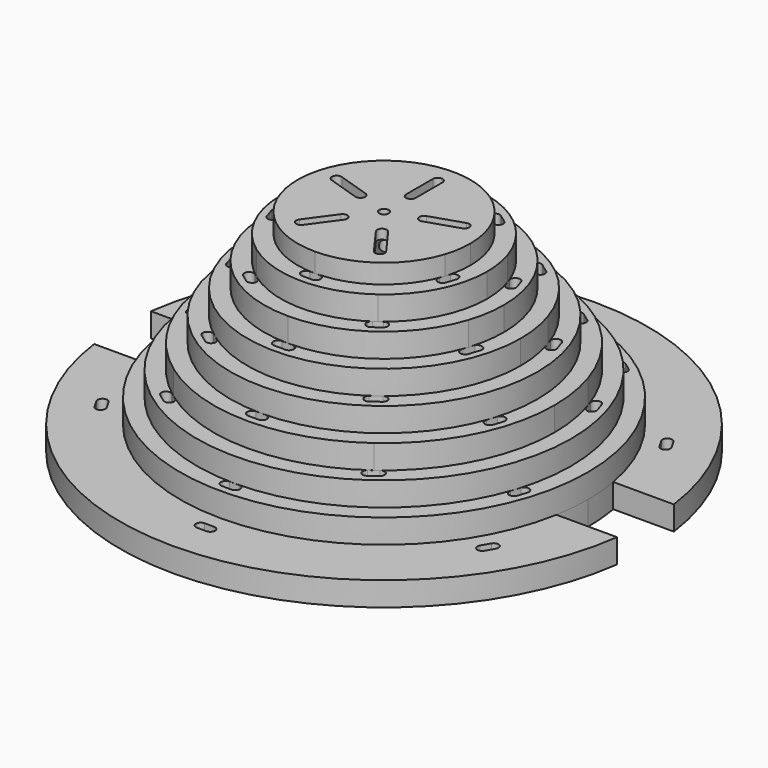
from build123d import *

# Parameters (mm, degrees)
F0_R      = 55
F1_DEPTH  = 5
F2_R      = 42.5
F3_DEPTH  = 5
F5_DEPTH  = 10.001
F7_DEPTH  = 5.001
F8_R      = 39
F9_DEPTH  = 5
F11_DEPTH = 15.001
F13_DEPTH = 5
F15_DEPTH = 20.001
F16_R     = 32
F17_DEPTH = 5
F19_DEPTH = 5
F21_DEPTH = 30.001
F22_DEPTH = 20.001
F24_DEPTH = 5
F26_DEPTH = 35.001
F28_DEPTH = 5
F30_DEPTH = 40.001
F32_DEPTH = 4
F33_R     = 1
F34_DEPTH = 44.001
F41_DEPTH = 5.0010001


with BuildPart() as f1:
    # F0 (on Top) → F1 (new body)
    with BuildSketch(Plane.XY):
        Circle(F0_R)
    extrude(amount=F1_DEPTH)

    # F2 (on face) → F3 (join)
    with BuildSketch(Plane.XY.offset(5)):
        Circle(F2_R)
    extrude(amount=F3_DEPTH)

    # F4 (on face) → F5 (cut, through all)
    with BuildSketch(Plane.XY.offset(10)):
        with BuildLine():
            Line((1, -39), (-1, -39))
            ThreePointArc((-1, -39), (-2, -40), (-1, -41))
            Line((-1, -41), (1, -41))
            ThreePointArc((1, -41), (2, -40), (1, -39))
        make_face()
        with BuildLine():
            Line((37.4002211299, -11.1006062643), (36.7821871411, -13.0027192969))
            ThreePointArc((36.7821871411, -13.0027192969), (37.4242266631, -14.2627928076), (38.6843001737, -13.6207532857))
            Line((38.6843001737, -13.6207532857), (39.3023341625, -11.7186402531))
            ThreePointArc((39.3023341625, -11.7186402531), (38.6602946406, -10.4585667424), (37.4002211299, -11.1006062643))
        make_face()
        with BuildLine():
            Line((22.114607845, 32.1394480329), (23.7326418338, 30.9638775283))
            ThreePointArc((23.7326418338, 30.9638775283), (25.1294440804, 31.1851092704), (24.9082123384, 32.5819115171))
            Line((24.9082123384, 32.5819115171), (23.2901783496, 33.7574820217))
            ThreePointArc((23.2901783496, 33.7574820217), (21.8933761029, 33.5362502796), (22.114607845, 32.1394480329))
        make_face()
        with BuildLine():
            Line((-23.7326418338, 30.9638775283), (-22.114607845, 32.1394480329))
            ThreePointArc((-22.114607845, 32.1394480329), (-21.8933761029, 33.5362502796), (-23.2901783496, 33.7574820217))
            Line((-23.2901783496, 33.7574820217), (-24.9082123384, 32.5819115171))
            ThreePointArc((-24.9082123384, 32.5819115171), (-25.1294440804, 31.1851092704), (-23.7326418338, 30.9638775283))
        make_face()
        with BuildLine():
            Line((-36.7821871411, -13.0027192969), (-37.4002211299, -11.1006062643))
            ThreePointArc((-37.4002211299, -11.1006062643), (-38.6602946406, -10.4585667424), (-39.3023341625, -11.7186402531))
            Line((-39.3023341625, -11.7186402531), (-38.6843001737, -13.6207532857))
            ThreePointArc((-38.6843001737, -13.6207532857), (-37.4242266631, -14.2627928076), (-36.7821871411, -13.0027192969))
        make_face()
    extrude(amount=-F5_DEPTH, mode=Mode.SUBTRACT)

    # F6 (on face) → F7 (cut, through all)
    with BuildSketch(Plane.XY.offset(5)):
        with BuildLine():
            ThreePointArc((-1, 47.5), (-2, 46.5), (-1, 45.5))
            Line((-1, 45.5), (1, 45.5))
            ThreePointArc((1, 45.5), (2, 46.5), (1, 47.5))
            Line((1, 47.5), (-1, 47.5))
        make_face()
        with BuildLine():
            Line((-40.6362066798, 24.6160254038), (-41.6362066798, 22.8839745962))
            ThreePointArc((-41.6362066798, 22.8839745962), (-41.270181276, 21.5179491924), (-39.9041558722, 21.8839745962))
            Line((-39.9041558722, 21.8839745962), (-38.9041558722, 23.6160254038))
            ThreePointArc((-38.9041558722, 23.6160254038), (-39.270181276, 24.9820508076), (-40.6362066798, 24.6160254038))
        make_face()
        with BuildLine():
            Line((-41.6362066798, -22.8839745962), (-40.6362066798, -24.6160254038))
            ThreePointArc((-40.6362066798, -24.6160254038), (-39.270181276, -24.9820508076), (-38.9041558722, -23.6160254038))
            Line((-38.9041558722, -23.6160254038), (-39.9041558722, -21.8839745962))
            ThreePointArc((-39.9041558722, -21.8839745962), (-41.270181276, -21.5179491924), (-41.6362066798, -22.8839745962))
        make_face()
        with BuildLine():
            Line((-1, -47.5), (1, -47.5))
            ThreePointArc((1, -47.5), (2, -46.5), (1, -45.5))
            Line((1, -45.5), (-1, -45.5))
            ThreePointArc((-1, -45.5), (-2, -46.5), (-1, -47.5))
        make_face()
        with BuildLine():
            Line((40.6362066798, -24.6160254038), (41.6362066798, -22.8839745962))
            ThreePointArc((41.6362066798, -22.8839745962), (41.270181276, -21.5179491924), (39.9041558722, -21.8839745962))
            Line((39.9041558722, -21.8839745962), (38.9041558722, -23.6160254038))
            ThreePointArc((38.9041558722, -23.6160254038), (39.270181276, -24.9820508076), (40.6362066798, -24.6160254038))
        make_face()
        with BuildLine():
            Line((41.6362066798, 22.8839745962), (40.6362066798, 24.6160254038))
            ThreePointArc((40.6362066798, 24.6160254038), (39.270181276, 24.9820508076), (38.9041558722, 23.6160254038))
            Line((38.9041558722, 23.6160254038), (39.9041558722, 21.8839745962))
            ThreePointArc((39.9041558722, 21.8839745962), (41.270181276, 21.5179491924), (41.6362066798, 22.8839745962))
        make_face()
    extrude(amount=-F7_DEPTH, mode=Mode.SUBTRACT)

    # F8 (on face) → F9 (join)
    with BuildSketch(Plane.XY.offset(10)):
        Circle(F8_R)
    extrude(amount=F9_DEPTH)

    # F10 (on face) → F11 (cut, through all)
    with BuildSketch(Plane.XY.offset(15)):
        with BuildLine():
            ThreePointArc((1, 35.5), (2, 36.5), (1, 37.5))
            Line((1, 37.5), (-1, 37.5))
            ThreePointArc((-1, 37.5), (-2, 36.5), (-1, 35.5))
            Line((-1, 35.5), (1, 35.5))
        make_face()
        with BuildLine():
            ThreePointArc((-33.4534893341, 11.9211598166), (-34.095528856, 13.1812333273), (-35.3556023667, 12.5391938054))
            Line((-35.3556023667, 12.5391938054), (-35.9736363554, 10.6370807728))
            ThreePointArc((-35.9736363554, 10.6370807728), (-35.3315968335, 9.3770072621), (-34.0715233229, 10.019046784))
            Line((-34.0715233229, 10.019046784), (-33.4534893341, 11.9211598166))
        make_face()
        with BuildLine():
            ThreePointArc((-21.6753934508, -28.132318048), (-23.0721956974, -28.3535497901), (-22.8509639553, -29.7503520368))
            Line((-22.8509639553, -29.7503520368), (-21.2329299666, -30.9259225414))
            ThreePointArc((-21.2329299666, -30.9259225414), (-19.8361277199, -30.7046907993), (-20.057359462, -29.3078885526))
            Line((-20.057359462, -29.3078885526), (-21.6753934508, -28.132318048))
        make_face()
        with BuildLine():
            ThreePointArc((20.057359462, -29.3078885526), (19.8361277199, -30.7046907993), (21.2329299666, -30.9259225414))
            Line((21.2329299666, -30.9259225414), (22.8509639553, -29.7503520368))
            ThreePointArc((22.8509639553, -29.7503520368), (23.0721956974, -28.3535497901), (21.6753934508, -28.132318048))
            Line((21.6753934508, -28.132318048), (20.057359462, -29.3078885526))
        make_face()
        with BuildLine():
            ThreePointArc((34.0715233229, 10.019046784), (35.3315968335, 9.3770072621), (35.9736363554, 10.6370807728))
            Line((35.9736363554, 10.6370807728), (35.3556023667, 12.5391938054))
            ThreePointArc((35.3556023667, 12.5391938054), (34.095528856, 13.1812333273), (33.4534893341, 11.9211598166))
            Line((33.4534893341, 11.9211598166), (34.0715233229, 10.019046784))
        make_face()
    extrude(amount=-F11_DEPTH, mode=Mode.SUBTRACT)

    # F12 (on face) → F13 (join)
    with BuildSketch(Plane.XY.offset(15)):
        with BuildLine():
            ThreePointArc((20.8663763999, -28.7201033414), (31.6307315928, -16.1166627719), (35.5, 0))
            ThreePointArc((35.5, 0), (35.0629360728, 5.5534236244), (33.7625062562, 10.9701035227))
            ThreePointArc((33.7625062562, 10.9701035227), (20.8663763618, 28.720103369), (0, 35.5))
            ThreePointArc((0, 35.5), (-20.8663763618, 28.720103369), (-33.7625062562, 10.9701035227))
            ThreePointArc((-33.7625062562, 10.9701035227), (-33.7625063538, -10.9701032224), (-20.8663763999, -28.7201033414))
            ThreePointArc((-20.8663763999, -28.7201033414), (0, -35.5), (20.8663763999, -28.7201033414))
        make_face()
    extrude(amount=F13_DEPTH)

    # F14 (on face) → F15 (cut, through all)
    with BuildSketch(Plane.XY.offset(20)):
        with BuildLine():
            ThreePointArc((0.9018983435, -34), (2, -33.0981016565), (1.0981016565, -32))
            Line((1.0981016565, -32), (-1.0981016565, -32))
            ThreePointArc((-1.0981016565, -32), (-2.0981016565, -33), (-1.0981016565, -34))
            Line((-1.0981016565, -34), (0.9018983435, -34))
        make_face()
        with BuildLine():
            ThreePointArc((32.6146234694, -9.6488215121), (32.0961992461, -8.3257628608), (30.7731405948, -8.8441870841))
            Line((30.7731405948, -8.8441870841), (30.094476448, -10.9329005559))
            ThreePointArc((30.094476448, -10.9329005559), (30.73651597, -12.1929740666), (31.9965894806, -11.5509345447))
            Line((31.9965894806, -11.5509345447), (32.6146234694, -9.6488215121))
        make_face()
        with BuildLine():
            ThreePointArc((19.2550474908, 28.0367003541), (17.8365420438, 27.9524972262), (17.9207451717, 26.5339917792))
            Line((17.9207451717, 26.5339917792), (19.697510975, 25.2430958608))
            ThreePointArc((19.697510975, 25.2430958608), (21.0943132217, 25.4643276029), (20.8730814796, 26.8611298496))
            Line((20.8730814796, 26.8611298496), (19.2550474908, 28.0367003541))
        make_face()
        with BuildLine():
            ThreePointArc((-20.7143496651, 26.9764552634), (-21.0726100213, 25.6013562171), (-19.697510975, 25.2430958608))
            Line((-19.697510975, 25.2430958608), (-17.9207451717, 26.5339917792))
            ThreePointArc((-17.9207451717, 26.5339917792), (-17.6995134296, 27.9307940259), (-19.0963156763, 28.1520257679))
            Line((-19.0963156763, 28.1520257679), (-20.7143496651, 26.9764552634))
        make_face()
        with BuildLine():
            ThreePointArc((-32.0572196387, -11.3643341054), (-30.8601312686, -12.129988926), (-30.094476448, -10.9329005559))
            Line((-30.094476448, -10.9329005559), (-30.7731405948, -8.8441870841))
            ThreePointArc((-30.7731405948, -8.8441870841), (-32.0332141055, -8.2021475621), (-32.6752536274, -9.4622210728))
            Line((-32.6752536274, -9.4622210728), (-32.0572196387, -11.3643341054))
        make_face()
    extrude(amount=-F15_DEPTH, mode=Mode.SUBTRACT)

    # F16 (on face) → F17 (join)
    with BuildSketch(Plane.XY.offset(20)):
        Circle(F16_R)
        with BuildLine():
            ThreePointArc((-15.8373506425, -23.721428586), (-15.6161189004, -25.1182308327), (-17.0129211471, -25.3394625748))
            Line((-17.0129211471, -25.3394625748), (-18.6309551359, -24.1638920702))
            ThreePointArc((-18.6309551359, -24.1638920702), (-19.0343579254, -22.7959428829), (-17.6664087381, -22.3925400934))
            Line((-17.6664087381, -22.3925400934), (-15.8373506425, -23.721428586))
        make_face(mode=Mode.SUBTRACT)
        with BuildLine():
            ThreePointArc((17.6664087381, -22.3925400934), (19.0632109848, -22.6137718354), (18.8419792427, -24.0105740821))
            Line((18.8419792427, -24.0105740821), (17.223945254, -25.1861445867))
            ThreePointArc((17.223945254, -25.1861445867), (15.7982899479, -25.1470838921), (15.8373506425, -23.721428586))
            Line((15.8373506425, -23.721428586), (17.6664087381, -22.3925400934))
        make_face(mode=Mode.SUBTRACT)
        with BuildLine():
            ThreePointArc((-27.454429727, 7.7318909655), (-28.7145032376, 7.0898514436), (-29.3565427596, 8.3499249542))
            Line((-29.3565427596, 8.3499249542), (-28.7385087708, 10.2520379868))
            ThreePointArc((-28.7385087708, 10.2520379868), (-27.5621700999, 11.0584163848), (-26.7557917018, 9.8820777139))
            Line((-26.7557917018, 9.8820777139), (-27.454429727, 7.7318909655))
        make_face(mode=Mode.SUBTRACT)
        with BuildLine():
            Line((-1.1304200705, 30.5), (0.8695799295, 30.5))
            ThreePointArc((0.8695799295, 30.5), (2, 29.6304200705), (1.1304200705, 28.5))
            Line((1.1304200705, 28.5), (-1.1304200705, 28.5))
            ThreePointArc((-1.1304200705, 28.5), (-2.1304200705, 29.5), (-1.1304200705, 30.5))
        make_face(mode=Mode.SUBTRACT)
        with BuildLine():
            ThreePointArc((26.7557917018, 9.8820777139), (27.3978312238, 11.1421512245), (28.6579047344, 10.5001117026))
            Line((28.6579047344, 10.5001117026), (29.2759387232, 8.59799867))
            ThreePointArc((29.2759387232, 8.59799867), (28.7982380774, 7.2541903197), (27.454429727, 7.7318909655))
            Line((27.454429727, 7.7318909655), (26.7557917018, 9.8820777139))
        make_face(mode=Mode.SUBTRACT)
    extrude(amount=F17_DEPTH)

    # F18 (on face) → F19 (join)
    with BuildSketch(Plane.XY.offset(25)):
        with BuildLine():
            ThreePointArc((16.751879483, -23.0569844903), (25.3936858812, -12.9387293567), (28.5, 0))
            ThreePointArc((28.5, 0), (28.1491177387, 4.458382053), (27.1051108399, 8.8069839534))
            ThreePointArc((27.1051108399, 8.8069839534), (16.7518798547, 23.0569842203), (0, 28.5))
            ThreePointArc((0, 28.5), (-16.7518798298, 23.0569842384), (-27.1051108209, 8.8069840118))
            ThreePointArc((-27.1051108209, 8.8069840118), (-27.1051106855, -8.8069844287), (-16.7518798178, -23.0569842471))
            ThreePointArc((-16.7518798178, -23.0569842471), (-2.069e-07, -28.5), (16.751879483, -23.0569844903))
        make_face()
    extrude(amount=F19_DEPTH)

    # F20 (on face) → F21 (cut, through all)
    with BuildSketch(Plane.XY.offset(30)):
        with BuildLine():
            ThreePointArc((0.7057068686, -27), (2, -26.2942931314), (1.2942931314, -25))
            Line((1.2942931314, -25), (-1.2942931314, -25))
            ThreePointArc((-1.2942931314, -25), (-2.2942931314, -26), (-1.2942931314, -27))
            Line((-1.2942931314, -27), (0.7057068686, -27))
        make_face()
        with BuildLine():
            Line((24.1763714807, -6.4944789427), (23.3764543341, -8.956370776))
            ThreePointArc((23.3764543341, -8.956370776), (24.018493856, -10.2164442867), (25.2785673666, -9.5744047648))
            Line((25.2785673666, -9.5744047648), (25.8966013554, -7.6722917322))
            ThreePointArc((25.8966013554, -7.6722917322), (25.6253928128, -6.2232704001), (24.1763714807, -6.4944789427))
        make_face()
        with BuildLine():
            Line((13.6475261683, 20.9861912742), (15.7417364464, 19.4646584446))
            ThreePointArc((15.7417364464, 19.4646584446), (17.138538693, 19.6858901866), (16.9173069509, 21.0826924333))
            Line((16.9173069509, 21.0826924333), (15.2992729622, 22.2582629379))
            ThreePointArc((15.2992729622, 22.2582629379), (13.8373637334, 22.448100503), (13.6475261683, 20.9861912742))
        make_face()
        with BuildLine():
            Line((-15.7417364464, 19.4646584446), (-13.6475261683, 20.9861912742))
            ThreePointArc((-13.6475261683, 20.9861912742), (-13.4262944262, 22.3829935208), (-14.8230966729, 22.6042252629))
            Line((-14.8230966729, 22.6042252629), (-16.4411306616, 21.4286547583))
            ThreePointArc((-16.4411306616, 21.4286547583), (-17.0734317109, 20.0969594938), (-15.7417364464, 19.4646584446))
        make_face()
        with BuildLine():
            Line((-23.3764543341, -8.956370776), (-24.1763714807, -6.4944789427))
            ThreePointArc((-24.1763714807, -6.4944789427), (-25.4364449914, -5.8524394208), (-26.0784845133, -7.1125129315))
            Line((-26.0784845133, -7.1125129315), (-25.4604505245, -9.0146259641))
            ThreePointArc((-25.4604505245, -9.0146259641), (-24.3893248353, -10.0274964653), (-23.3764543341, -8.956370776))
        make_face()
    extrude(amount=-F21_DEPTH, mode=Mode.SUBTRACT)

    # F22 (cut, through all): faces of the model
    f22_faces = [f1.faces().sort_by_distance(p)[0] for p in [
        (17.3875864045, -23.8314304164, 20),
        (28.0380968803, 9.1722603537, 20),
        (-0.0590895526, 29.5001990686, 20),
        (-28.0746162322, 9.0598653456, 20),
        (-17.2919775, -23.9008943515, 20),
    ]]
    extrude(f22_faces, amount=-F22_DEPTH, mode=Mode.SUBTRACT)

    # F23 (on face) → F24 (join)
    with BuildSketch(Plane.XY.offset(30)):
        with BuildLine():
            ThreePointArc((23.7764129613, -7.7254246936), (24.6922085285, -3.9108615399), (25, 0))
            ThreePointArc((25, 0), (22.2751630699, 11.3497625618), (14.6946311833, 20.2254249495))
            ThreePointArc((14.6946311833, 20.2254249495), (-7.01e-08, 25), (-14.6946312967, 20.2254248671))
            ThreePointArc((-14.6946312967, 20.2254248671), (-23.7764128803, 7.7254249427), (-23.7764129574, -7.7254247053))
            ThreePointArc((-23.7764129574, -7.7254247053), (-14.6946313729, -20.2254248118), (0, -25))
            ThreePointArc((0, -25), (14.6946313778, -20.2254248081), (23.7764129613, -7.7254246936))
        make_face()
    extrude(amount=F24_DEPTH)

    # F25 (on face) → F26 (cut, through all)
    with BuildSketch(Plane.XY.offset(35)):
        with BuildLine():
            ThreePointArc((0.8893935699, 21.5), (2, 22.3893935699), (1.1106064301, 23.5))
            Line((1.1106064301, 23.5), (-0.8893935699, 23.5))
            ThreePointArc((-0.8893935699, 23.5), (-1.8893935699, 22.5), (-0.8893935699, 21.5))
            Line((-0.8893935699, 21.5), (0.8893935699, 21.5))
        make_face()
        with BuildLine():
            Line((-22.006631872, 8.3181488502), (-22.6246658607, 6.4160358176))
            ThreePointArc((-22.6246658607, 6.4160358176), (-21.9826263388, 5.1559623069), (-20.7225528281, 5.7980018289))
            Line((-20.7225528281, 5.7980018289), (-20.1728773726, 7.4897289293))
            ThreePointArc((-20.1728773726, 7.4897289293), (-20.6755446618, 8.8208161394), (-22.006631872, 8.3181488502))
        make_face()
        with BuildLine():
            Line((-14.7114529049, -18.3591012871), (-13.0934189161, -19.5346717917))
            ThreePointArc((-13.0934189161, -19.5346717917), (-11.6966166695, -19.3134400496), (-11.9178484115, -17.9166378029))
            Line((-11.9178484115, -17.9166378029), (-13.356917437, -16.8710929552))
            ThreePointArc((-13.356917437, -16.8710929552), (-14.7781893369, -16.9378293872), (-14.7114529049, -18.3591012871))
        make_face()
        with BuildLine():
            Line((12.9144539529, -19.6646974485), (14.5324879416, -18.4891269439))
            ThreePointArc((14.5324879416, -18.4891269439), (14.7537196837, -17.0923246973), (13.356917437, -16.8710929552))
            Line((13.356917437, -16.8710929552), (11.9178484115, -17.9166378029))
            ThreePointArc((11.9178484115, -17.9166378029), (11.5421213594, -19.2889703964), (12.9144539529, -19.6646974485))
        make_face()
        with BuildLine():
            Line((22.6930243939, 6.2056498854), (22.0749904051, 8.107762918))
            ThreePointArc((22.0749904051, 8.107762918), (20.8149168945, 8.7498024399), (20.1728773726, 7.4897289293))
            Line((20.1728773726, 7.4897289293), (20.7225528281, 5.7980018289))
            ThreePointArc((20.7225528281, 5.7980018289), (21.9116126393, 5.0165900743), (22.6930243939, 6.2056498854))
        make_face()
    extrude(amount=-F26_DEPTH, mode=Mode.SUBTRACT)

    # F27 (on face) → F28 (join)
    with BuildSketch(Plane.XY.offset(35)):
        with BuildLine():
            ThreePointArc((12.6373831456, -17.3938652183), (19.1566403321, -9.7607956226), (21.5, 0))
            ThreePointArc((21.5, 0), (21.2352993391, 3.3633408951), (20.447715165, 6.6438651802))
            ThreePointArc((20.447715165, 6.6438651802), (12.6373830089, 17.3938653176), (0, 21.5))
            ThreePointArc((0, 21.5), (-12.637382926, 17.3938653778), (-20.4477151017, 6.643865375))
            ThreePointArc((-20.4477151017, 6.643865375), (-20.447715142, -6.643865251), (-12.6373831456, -17.3938652183))
            ThreePointArc((-12.6373831456, -17.3938652183), (0, -21.5), (12.6373831456, -17.3938652183))
        make_face()
    extrude(amount=F28_DEPTH)

    # F29 (on face) → F30 (cut, through all)
    with BuildSketch(Plane.XY.offset(40)):
        with BuildLine():
            ThreePointArc((-1, 47.5), (-2, 46.5), (-1, 45.5))
            Line((-1, 45.5), (1, 45.5))
            ThreePointArc((1, 45.5), (2, 46.5), (1, 47.5))
            Line((1, 47.5), (-1, 47.5))
        make_face()
        with BuildLine():
            ThreePointArc((-1.069542788, -18), (-2.069542788, -19), (-1.069542788, -20))
            Line((-1.069542788, -20), (0.930457212, -20))
            ThreePointArc((0.930457212, -20), (2, -19.069542788), (1.069542788, -18))
            Line((1.069542788, -18), (-1.069542788, -18))
        make_face()
        with BuildLine():
            Line((17.449524191, -4.5451102608), (16.7885103956, -6.5795015367))
            ThreePointArc((16.7885103956, -6.5795015367), (17.4305499175, -7.8395750474), (18.6906234282, -7.1975355255))
            Line((18.6906234282, -7.1975355255), (19.308657417, -5.2954224929))
            ThreePointArc((19.308657417, -5.2954224929), (18.75424692, -3.9906997639), (17.449524191, -4.5451102608))
        make_face()
        with BuildLine():
            Line((9.7148562496, 15.1909673762), (11.4454128329, 13.9336444213))
            ThreePointArc((11.4454128329, 13.9336444213), (12.8422150796, 14.1548761634), (12.6209833375, 15.55167841))
            Line((12.6209833375, 15.55167841), (11.0029493488, 16.7272489146))
            ThreePointArc((11.0029493488, 16.7272489146), (9.59076203, 16.603154695), (9.7148562496, 15.1909673762))
        make_face()
        with BuildLine():
            Line((-11.4454128329, 13.9336444213), (-9.7148562496, 15.1909673762))
            ThreePointArc((-9.7148562496, 15.1909673762), (-9.4936245075, 16.5877696229), (-10.8904267542, 16.809001365))
            Line((-10.8904267542, 16.809001365), (-12.5084607429, 15.6334308604))
            ThreePointArc((-12.5084607429, 15.6334308604), (-12.8268300075, 14.2520136858), (-11.4454128329, 13.9336444213))
        make_face()
        with BuildLine():
            Line((-16.7885103956, -6.5795015367), (-17.449524191, -4.5451102608))
            ThreePointArc((-17.449524191, -4.5451102608), (-18.7095977017, -3.9030707389), (-19.3516372236, -5.1631442495))
            Line((-19.3516372236, -5.1631442495), (-18.7336032348, -7.0652572821))
            ThreePointArc((-18.7336032348, -7.0652572821), (-17.5181789425, -7.794925829), (-16.7885103956, -6.5795015367))
        make_face()
    extrude(amount=-F30_DEPTH, mode=Mode.SUBTRACT)

    # F31 (on face) → F32 (join)
    with BuildSketch(Plane.XY.offset(40)):
        with BuildLine():
            ThreePointArc((17.1190174208, -5.5623055065), (17.778390163, -2.815820167), (18, 0))
            ThreePointArc((18, 0), (16.0381174444, 8.1718289776), (10.5801345734, 14.5623058754))
            ThreePointArc((10.5801345734, 14.5623058754), (0, 18), (-10.5801345734, 14.5623058754))
            ThreePointArc((-10.5801345734, 14.5623058754), (-17.1190172092, 5.5623061575), (-17.1190174737, -5.5623053435))
            ThreePointArc((-17.1190174737, -5.5623053435), (-10.5801347774, -14.5623057272), (0, -18))
            ThreePointArc((0, -18), (10.5801347081, -14.5623057775), (17.1190174208, -5.5623055065))
        make_face()
    extrude(amount=F32_DEPTH)

    # F33 (on face) → F34 (cut, through all)
    with BuildSketch(Plane.XY.offset(44)):
        Circle(F33_R)
        with BuildLine():
            Line((-1, 14), (-1, 7))
            ThreePointArc((-1, 7), (0, 6), (1, 7))
            Line((1, 7), (1, 14))
            ThreePointArc((1, 14), (0, 15), (-1, 14))
        make_face()
        with BuildLine():
            Line((-6.3483786197, 3.1141754769), (-13.0057742338, 5.2772944375))
            ThreePointArc((-13.0057742338, 5.2772944375), (-14.2658477444, 4.6352549156), (-13.6238082225, 3.375181405))
            Line((-13.6238082225, 3.375181405), (-6.9664126084, 1.2120624443))
            ThreePointArc((-6.9664126084, 1.2120624443), (-5.7063390978, 1.8541019662), (-6.3483786197, 3.1141754769))
        make_face()
        with BuildLine():
            Line((-4.9235137604, -5.0753337083), (-9.0380105265, -10.738452669))
            ThreePointArc((-9.0380105265, -10.738452669), (-8.8167787844, -12.1352549156), (-7.4199765377, -11.9140231735))
            Line((-7.4199765377, -11.9140231735), (-3.3054797717, -6.2509042129))
            ThreePointArc((-3.3054797717, -6.2509042129), (-3.5267115138, -4.8541019662), (-4.9235137604, -5.0753337083))
        make_face()
        with BuildLine():
            Line((3.3054797717, -6.2509042129), (7.4199765377, -11.9140231735))
            ThreePointArc((7.4199765377, -11.9140231735), (8.8167787844, -12.1352549156), (9.0380105265, -10.738452669))
            Line((9.0380105265, -10.738452669), (4.9235137604, -5.0753337083))
            ThreePointArc((4.9235137604, -5.0753337083), (3.5267115138, -4.8541019662), (3.3054797717, -6.2509042129))
        make_face()
        with BuildLine():
            Line((6.9664126084, 1.2120624443), (13.6238082225, 3.375181405))
            ThreePointArc((13.6238082225, 3.375181405), (14.2658477444, 4.6352549156), (13.0057742338, 5.2772944375))
            Line((13.0057742338, 5.2772944375), (6.3483786197, 3.1141754769))
            ThreePointArc((6.3483786197, 3.1141754769), (5.7063390978, 1.8541019662), (6.9664126084, 1.2120624443))
        make_face()
    extrude(amount=-F34_DEPTH, mode=Mode.SUBTRACT)

    # F38 (on Right) → F39 (revolve, cut)
    with BuildSketch(Plane.YZ):
        Polygon((15, 42), (0, 42), (0, 0), (41, 0), align=None)
    revolve(axis=Axis((0, 0, 21), (0, 0, 1)), mode=Mode.SUBTRACT)

    # F40 (on face) → F41 (cut, through all)
    with BuildSketch(Plane.XY.offset(5)):
        with BuildLine():
            ThreePointArc((-41.8508064438, -7.4), (-42.5, 0), (-41.8508064438, 7.4))
            Line((-41.8508064438, 7.4), (-54.4999082568, 7.4))
            ThreePointArc((-54.4999082568, 7.4), (-55, 0), (-54.4999082568, -7.4))
            Line((-54.4999082568, -7.4), (-41.8508064438, -7.4))
        make_face()
        with BuildLine():
            Line((54.4999082568, 7.4), (41.8508064438, 7.4))
            ThreePointArc((41.8508064438, 7.4), (42.3373905305, 3.7142109617), (42.5, 0))
            ThreePointArc((42.5, 0), (42.3373905305, -3.7142109617), (41.8508064438, -7.4))
            Line((41.8508064438, -7.4), (54.4999082568, -7.4))
            ThreePointArc((54.4999082568, -7.4), (54.8748346427, -3.7084394208), (55, 0))
            ThreePointArc((55, 0), (54.8748346427, 3.7084394208), (54.4999082568, 7.4))
        make_face()
    extrude(amount=-F41_DEPTH, mode=Mode.SUBTRACT)


solid = f1.part
